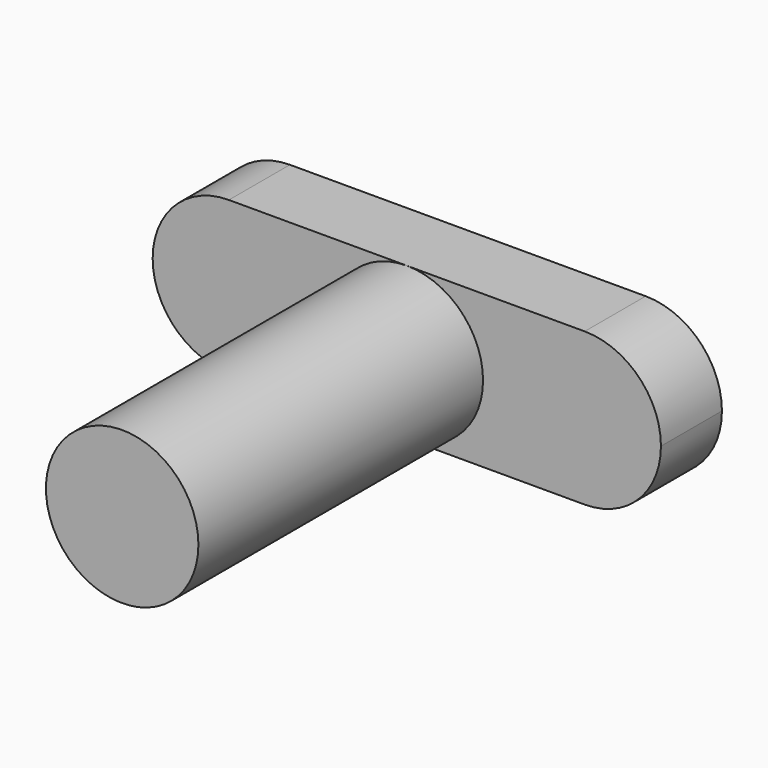
from build123d import *

# Parameters (mm, degrees)
F0_R     = 3
F1_DEPTH = 14
F3_DEPTH = 3


with BuildPart() as f1:
    # F0 (on Front) → F1 (new body)
    with BuildSketch(Plane.XZ):
        Circle(F0_R)
    extrude(amount=F1_DEPTH)

    # F2 (on face) → F3 (join)
    with BuildSketch(Plane(origin=(0, 0, 0), x_dir=(-1, 0, 0), z_dir=(0, 1, 0))):
        with BuildLine():
            ThreePointArc((-10, 0), (-9.1213203436, -2.1213203436), (-7, -3))
            Line((-7, -3), (0, -3))
            ThreePointArc((0, -3), (-3, 0), (0, 3))
            Line((0, 3), (-7, 3))
            ThreePointArc((-7, 3), (-9.1213203436, 2.1213203436), (-10, 0))
        make_face()
        with BuildLine():
            ThreePointArc((3, 0), (2.1213203436, -2.1213203436), (0, -3))
            Line((0, -3), (7, -3))
            ThreePointArc((7, -3), (9.1213203436, -2.1213203436), (10, 0))
            ThreePointArc((10, 0), (9.1213203436, 2.1213203436), (7, 3))
            Line((7, 3), (0, 3))
            ThreePointArc((0, 3), (2.1213203436, 2.1213203436), (3, 0))
        make_face()
        with BuildLine():
            ThreePointArc((0, 3), (-3, 0), (0, -3))
            ThreePointArc((0, -3), (2.1213203436, -2.1213203436), (3, 0))
            ThreePointArc((3, 0), (2.1213203436, 2.1213203436), (0, 3))
        make_face()
    extrude(amount=F3_DEPTH)


solid = f1.part
